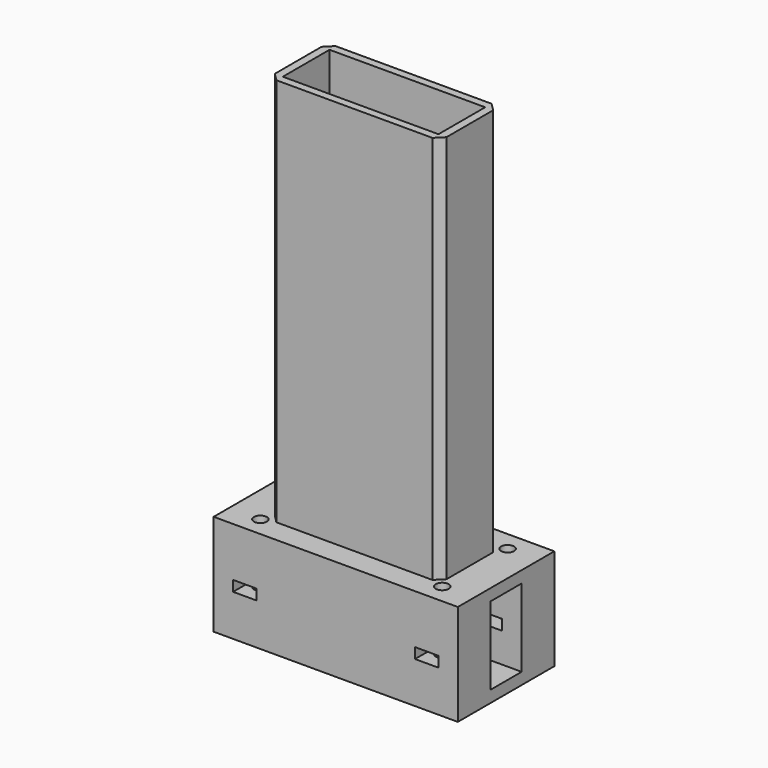
from build123d import *

# Parameters (mm, degrees)
F0_W     = 62.7378050089
F0_H     = 31
F0_W_2   = 40
F0_H_2   = 15
F1_DEPTH = 26
F2_W     = 10
F2_H     = 20
F3_DEPTH = 62.7388050089
F4_D     = 3.3
F5_W     = 44.1129240592
F5_H     = 19
F5_W_2   = 40
F5_H_2   = 15
F6_DEPTH = 100
F7_SIZE  = 2
F8_W     = 6
F8_H     = 2.7
F9_DEPTH = 31.001


with BuildPart() as f1:
    # F0 (on Top) → F1 (new body)
    with BuildSketch(Plane.XY):
        Rectangle(F0_W, F0_H)
        Rectangle(F0_W_2, F0_H_2, mode=Mode.SUBTRACT)
    extrude(amount=F1_DEPTH)

    # F2 (on face) → F3 (cut, through all)
    with BuildSketch(Plane(origin=(-31.3689025044, 0, 0), x_dir=(0, -1, 0), z_dir=(-1, 0, 0))):
        with Locations((0, 13)):
            Rectangle(F2_W, F2_H)
    extrude(amount=-F3_DEPTH, mode=Mode.SUBTRACT)

    # F4 (through all)
    with Locations(Plane(origin=(0, 0, 0), x_dir=(1, 0, 0), z_dir=(0, 0, -1))):
        with Locations((-23.3689025044, -10.5), (-23.3689025044, 10.5), (23.3689025044, 10.5), (23.3689025044, -10.5)):
            Hole(F4_D / 2)

    # F5 (on face) → F6 (join)
    with BuildSketch(Plane.XY.offset(26)):
        Rectangle(F5_W, F5_H)
        Rectangle(F5_W_2, F5_H_2, mode=Mode.SUBTRACT)
    extrude(amount=F6_DEPTH)

    # F7
    f7_edges = [f1.edges().sort_by_distance(p)[0] for p in [
        (22.056462, 9.5, 76),
        (-22.056462, 9.5, 76),
        (22.056462, -9.5, 76),
        (-22.056462, -9.5, 76),
    ]]
    chamfer(f7_edges, length=F7_SIZE)

    # F8 (on face) → F9 (cut, through all)
    with BuildSketch(Plane.XZ.offset(15.5)):
        with Locations((-23.3689025044, 12)):
            Rectangle(F8_W, F8_H)
        with Locations((23.3689025044, 12)):
            Rectangle(F8_W, F8_H)
    extrude(amount=-F9_DEPTH, mode=Mode.SUBTRACT)


solid = f1.part
